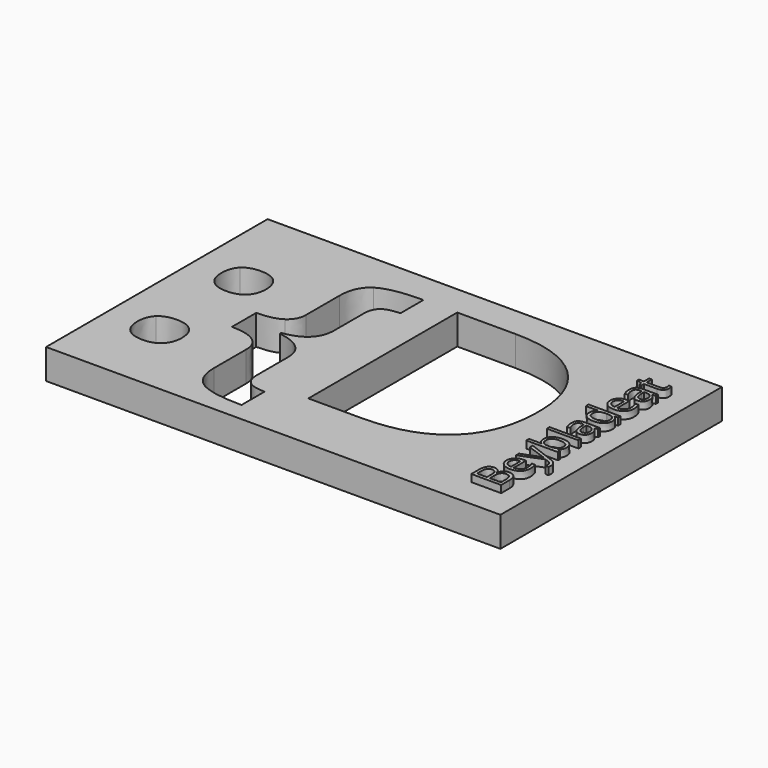
from build123d import *

# Parameters (mm, degrees)
F1_DEPTH     = 12.7
F2_TEXT_SIZE = 17.7036602205
F3_DEPTH     = 3.048


# Not quite as in the source:
# - Text() gives the source's letters only with a copy of the font that has no kerning and outlines rounded to 1/6400 em; it was checked with that copy


with BuildPart() as f1:
    # F0 (on Top) → F1 (new body)
    with BuildSketch(Plane.XY):
        Polygon((0, 0), (0, -12.7466353588), (192.4400627613, -12.7466353588), (192.4400627613, 0), (192.4400627613, 104.5206561685), (0, 104.5206561685), align=None)
        with BuildLine():
            add(Edge.make_bspline(
                [(14.6327171327, 13.607107147), (12.1568233678, 16.005359644), (12.1568233678, 20.3705242609)],
                knots=[0, 0, 0, 1, 1, 1], degree=2))
            add(Edge.make_bspline(
                [(12.1568233678, 20.3705242609), (12.1568233678, 24.8909714136), (14.5809562874, 27.2115826428)],
                knots=[0, 0, 0, 1, 1, 1], degree=2))
            add(Edge.make_bspline(
                [(14.5809562874, 27.2115826428), (17.0050892071, 29.5321938719), (21.6463116654, 29.5321938719)],
                knots=[0, 0, 0, 1, 1, 1], degree=2))
            add(Edge.make_bspline(
                [(21.6463116654, 29.5321938719), (26.1149979728, 29.5321938719), (28.5650113151, 27.1598217975)],
                knots=[0, 0, 0, 1, 1, 1], degree=2))
            add(Edge.make_bspline(
                [(28.5650113151, 27.1598217975), (31.0150246574, 24.7874497231), (31.0150246574, 20.3705242609)],
                knots=[0, 0, 0, 1, 1, 1], degree=2))
            add(Edge.make_bspline(
                [(31.0150246574, 20.3705242609), (31.0150246574, 16.1088813345), (28.5391308925, 13.6588679922)],
                knots=[0, 0, 0, 1, 1, 1], degree=2))
            add(Edge.make_bspline(
                [(28.5391308925, 13.6588679922), (26.0632371276, 11.2088546499), (21.6463116654, 11.2088546499)],
                knots=[0, 0, 0, 1, 1, 1], degree=2))
            add(Edge.make_bspline(
                [(21.6463116654, 11.2088546499), (17.1086108976, 11.2088546499), (14.6327171327, 13.607107147)],
                knots=[0, 0, 0, 1, 1, 1], degree=2))
        make_face(mode=Mode.SUBTRACT)
        with BuildLine():
            Line((52.8063405118, 10.22539859), (52.8063405118, 27.2202094503))
            add(Edge.make_bspline(
                [(52.8063405118, 27.2202094503), (52.8063405118, 31.9131927539), (49.2779762266, 34.3890865188)],
                knots=[0, 0, 0, 1, 1, 1], degree=2))
            add(Edge.make_bspline(
                [(49.2779762266, 34.3890865188), (45.7496119414, 36.8649802837), (39.0034484425, 36.8649802837)],
                knots=[0, 0, 0, 1, 1, 1], degree=2))
            Line((39.0034484425, 36.8649802837), (39.0034484425, 49.7534307534))
            add(Edge.make_bspline(
                [(39.0034484425, 49.7534307534), (45.8013727867, 49.7534307534), (49.3038566492, 52.1258028279)],
                knots=[0, 0, 0, 1, 1, 1], degree=2))
            add(Edge.make_bspline(
                [(49.3038566492, 52.1258028279), (52.8063405118, 54.4981749023), (52.8063405118, 58.9151003644)],
                knots=[0, 0, 0, 1, 1, 1], degree=2))
            Line((52.8063405118, 58.9151003644), (52.8063405118, 59.3464407416))
            Line((52.8063405118, 59.3464407416), (52.8063405118, 76.4965341377))
            add(Edge.make_bspline(
                [(52.8063405118, 76.4965341377), (52.8063405118, 84.7437621491), (58.0341858831, 88.1168438985)],
                knots=[0, 0, 0, 1, 1, 1], degree=2))
            add(Edge.make_bspline(
                [(58.0341858831, 88.1168438985), (63.2620312543, 91.489925648), (76.4265395654, 91.489925648)],
                knots=[0, 0, 0, 1, 1, 1], degree=2))
            Line((76.4265395654, 91.489925648), (76.4265395654, 79.3606342421))
            add(Edge.make_bspline(
                [(76.4265395654, 79.3606342421), (71.0779188886, 79.1880980912), (69.0592459234, 77.3074540468)],
                knots=[0, 0, 0, 1, 1, 1], degree=2))
            add(Edge.make_bspline(
                [(69.0592459234, 77.3074540468), (67.0405729583, 75.4268100023), (67.0405729583, 71.7517899889)],
                knots=[0, 0, 0, 1, 1, 1], degree=2))
            Line((67.0405729583, 71.7517899889), (67.0405729583, 55.636913498))
            add(Edge.make_bspline(
                [(67.0405729583, 55.636913498), (66.7127542716, 45.491787827), (54.42818033, 43.6629046279)],
                knots=[0, 0, 0, 1, 1, 1], degree=2))
            Line((54.42818033, 43.6629046279), (54.42818033, 43.0072672546))
            add(Edge.make_bspline(
                [(54.42818033, 43.0072672546), (67.0405729583, 41.1266232101), (67.0405729583, 31.5853740672)],
                knots=[0, 0, 0, 1, 1, 1], degree=2))
            Line((67.0405729583, 31.5853740672), (67.0405729583, 31.1022728448))
            Line((67.0405729583, 31.1022728448), (67.0405729583, 14.9701427388))
            add(Edge.make_bspline(
                [(67.0405729583, 14.9701427388), (67.0405729583, 11.3123763405), (69.0333655008, 9.4231054885)],
                knots=[0, 0, 0, 1, 1, 1], degree=2))
            add(Edge.make_bspline(
                [(69.0333655008, 9.4231054885), (71.0261580433, 7.5338346365), (76.4265395654, 7.3785521007)],
                knots=[0, 0, 0, 1, 1, 1], degree=2))
            Line((76.4265395654, 7.3785521007), (76.4265395654, -4.8197537655))
            add(Edge.make_bspline(
                [(76.4265395654, -4.8197537655), (63.2620312543, -4.8197537655), (58.0341858831, -1.4466720161)],
                knots=[0, 0, 0, 1, 1, 1], degree=2))
            add(Edge.make_bspline(
                [(58.0341858831, -1.4466720161), (52.8063405118, 1.9264097333), (52.8063405118, 10.22539859)],
                knots=[0, 0, 0, 1, 1, 1], degree=2))
        make_face(mode=Mode.SUBTRACT)
        with BuildLine():
            add(Edge.make_bspline(
                [(14.6327171327, 58.1128072629), (12.1568233678, 60.4851793373), (12.1568233678, 64.9021047995)],
                knots=[0, 0, 0, 1, 1, 1], degree=2))
            add(Edge.make_bspline(
                [(12.1568233678, 64.9021047995), (12.1568233678, 69.4398055673), (14.5809562874, 71.7517899889)],
                knots=[0, 0, 0, 1, 1, 1], degree=2))
            add(Edge.make_bspline(
                [(14.5809562874, 71.7517899889), (17.0050892071, 74.0637744105), (21.6463116654, 74.0637744105)],
                knots=[0, 0, 0, 1, 1, 1], degree=2))
            add(Edge.make_bspline(
                [(21.6463116654, 74.0637744105), (26.1149979728, 74.0637744105), (28.5650113151, 71.6914023361)],
                knots=[0, 0, 0, 1, 1, 1], degree=2))
            add(Edge.make_bspline(
                [(28.5650113151, 71.6914023361), (31.0150246574, 69.3190302617), (31.0150246574, 64.9021047995)],
                knots=[0, 0, 0, 1, 1, 1], degree=2))
            add(Edge.make_bspline(
                [(31.0150246574, 64.9021047995), (31.0150246574, 60.5369401826), (28.5132504699, 58.1386876855)],
                knots=[0, 0, 0, 1, 1, 1], degree=2))
            add(Edge.make_bspline(
                [(28.5132504699, 58.1386876855), (26.0114762823, 55.7404351885), (21.6463116654, 55.7404351885)],
                knots=[0, 0, 0, 1, 1, 1], degree=2))
            add(Edge.make_bspline(
                [(21.6463116654, 55.7404351885), (17.1086108976, 55.7404351885), (14.6327171327, 58.1128072629)],
                knots=[0, 0, 0, 1, 1, 1], degree=2))
        make_face(mode=Mode.SUBTRACT)
        with BuildLine():
            add(Edge.make_bspline(
                [(145.4927607572, 81.3016659393), (156.1727484958, 71.1134062307), (156.1727484958, 52.8245742389)],
                knots=[0, 0, 0, 1, 1, 1], degree=2))
            add(Edge.make_bspline(
                [(156.1727484958, 52.8245742389), (156.1727484958, 33.3624964212), (145.0873008026, 23.0103273692)],
                knots=[0, 0, 0, 1, 1, 1], degree=2))
            add(Edge.make_bspline(
                [(145.0873008026, 23.0103273692), (134.0018531095, 12.6581583172), (113.0904716245, 12.6581583172)],
                knots=[0, 0, 0, 1, 1, 1], degree=2))
            Line((113.0904716245, 12.6581583172), (90.7642937024, 12.6581583172))
            Line((90.7642937024, 12.6581583172), (90.7642937024, 91.489925648))
            Line((90.7642937024, 91.489925648), (115.5059777366, 91.489925648))
            add(Edge.make_bspline(
                [(115.5059777366, 91.489925648), (134.8127730185, 91.489925648), (145.4927607572, 81.3016659393)],
                knots=[0, 0, 0, 1, 1, 1], degree=2))
        make_face(mode=Mode.SUBTRACT)
    extrude(amount=F1_DEPTH)

    # F2 (on face) → F3 (join)
    with BuildSketch(Plane.XY.offset(12.7)):
        with Locations(Location((182.9482018948, -2.2295116382), (0, 0, 90))):
            Text('Beybladeat', F2_TEXT_SIZE, font='Open Sans', text_align=(TextAlign.LEFT, TextAlign.BOTTOM))
    extrude(amount=F3_DEPTH)


solid = f1.part
